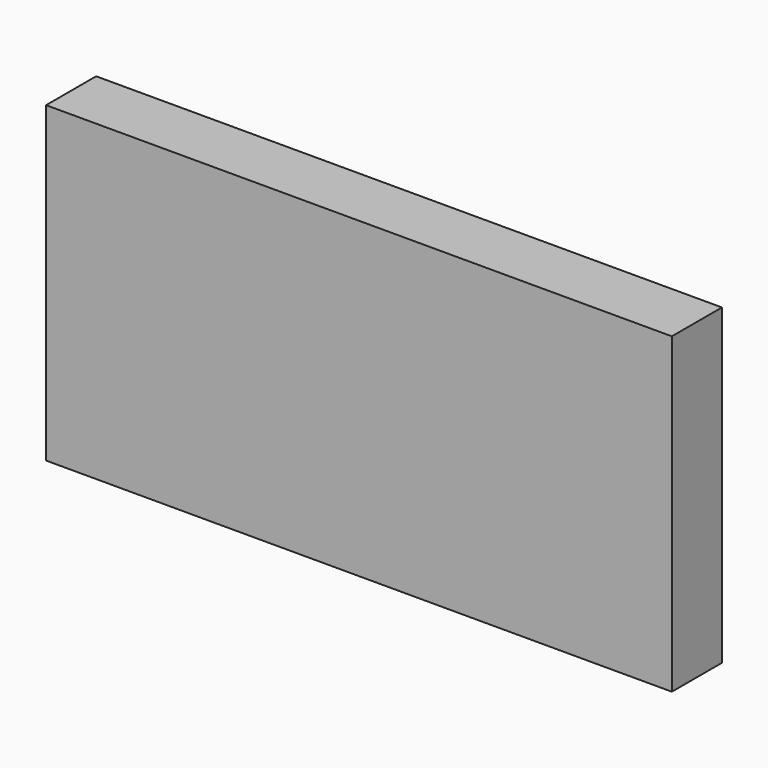
from build123d import *

# Parameters (mm, degrees)
F1_W     = 1270
F1_H     = 635
F2_DEPTH = 127


# Not quite as in the source:
# - a variable given as a bare number and used for a length is read in inches; the dataset says mm whatever the document's units were


with BuildPart() as f2:
    # F1 (on Front) → F2 (new body)
    with BuildSketch(Plane.XZ):
        with Locations((-635, 317.5)):
            Rectangle(F1_W, F1_H)
    extrude(amount=F2_DEPTH)


solid = f2.part
